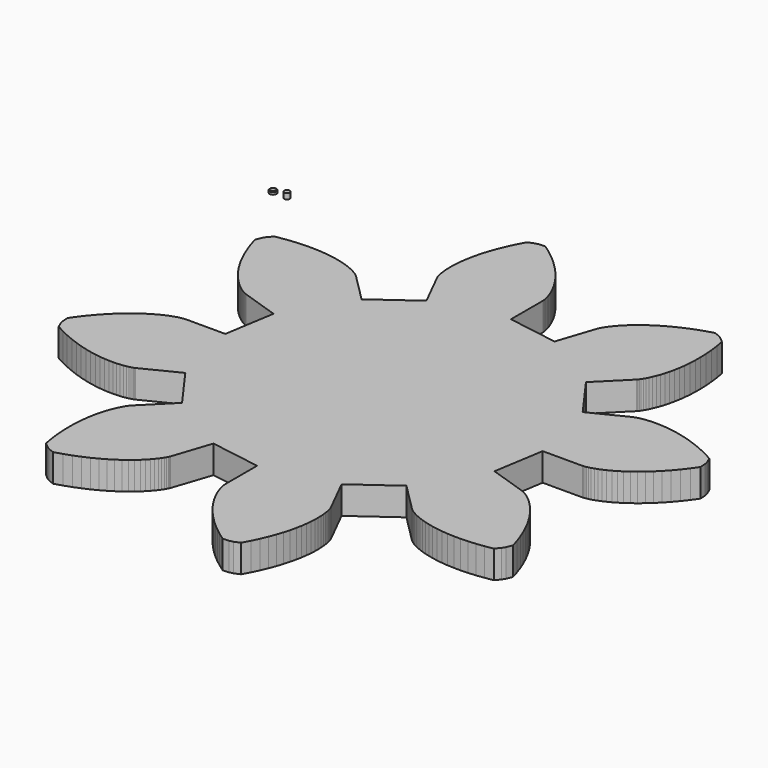
from build123d import *

# Parameters (mm, degrees)
F0_R     = 31.75
F0_R_2   = 25.4
F1_DEPTH = 25.4
F0_R_3   = 25.4571162214
F2_DEPTH = 50.8
F3_R     = 2.54
F6_DEPTH = 254


# Not quite as in the source:
# - a fillet or chamfer that OpenCascade refuses, or shapes differently, is made with other operations: its cross-section is extruded or revolved along the edge and cut away or added


with BuildPart() as f1:
    # F0 (on Top) → F1 (new body)
    with BuildSketch(Plane.XY):
        with Locations((-25.4, 10.8899995685)):
            Circle(F0_R)
        with Locations((-25.4, 10.8899995685)):
            Circle(F0_R_2, mode=Mode.SUBTRACT)
    extrude(amount=F1_DEPTH)

    # F3
    f3_edges = [f1.edges().sort_by_distance(p)[0] for p in [
        (-50.8, 10.89, 25.4),
    ]]
    fillet(f3_edges, radius=F3_R)

    # F4: chamfer of 5.08 on 1 edges, made by hand

    # F4_s1 → F4_t2 (revolve, cut)
    with BuildSketch(Plane.XZ.offset(-10.8899995685)):
        Polygon((1.27, 25.4), (6.35, 20.32), (6.35, 25.4), align=None)
    revolve(axis=Axis((-25.4, 10.8899995685, 25.4), (0, 0, 1)), mode=Mode.SUBTRACT)


with BuildPart() as f2:
    # F0 (on Top) → F2 (new body)
    with BuildSketch(Plane.XY):
        with Locations((101.6, 10.8899995685)):
            Circle(F0_R_3)
    extrude(amount=F2_DEPTH)


with BuildPart() as f6:
    # F5 (on face) → F6 (new body)
    with BuildSketch(Plane.XY.offset(50.8)):
        Polygon((4697.3145576, -2359.8523288), (4703.8413416, -2359.2975928), (4713.7554696, -2358.0235288), (4727.0000456, -2355.7354968), (4743.5019176, -2352.1408888), (4763.1635496, -2346.9511608), (4785.8731816, -2339.8858968), (4811.4967016, -2330.6728088), (4839.8837416, -2319.0457048), (4870.8656456, -2304.7485528), (4904.2595336, -2287.5354808), (4939.8642376, -2267.1728088), (4977.4603016, -2243.4349848), (5016.8181096, -2216.1167768), (5057.6897576, -2185.0210808), (5099.8151496, -2149.9690808), (5142.9240296, -2110.7941528), (5186.7319176, -2067.3520248), (5230.9421416, -2019.5065528), (5275.2499016, -1967.1480088), (5319.3422696, -1910.1829208), (5362.8961576, -1848.5340728), (5359.2670056, -1792.7556728), (5351.1227496, -1758.3092088), (5329.3864456, -1706.8142648), (5262.8323496, -1671.1994008), (5197.8977576, -1640.0122648), (5134.8326056, -1613.0435608), (5073.8766696, -1590.0657048), (5015.2514376, -1570.8429848), (4959.1641736, -1555.1234328), (4905.7997896, -1542.6489848), (4855.3289736, -1533.1514168), (4807.9041256, -1526.3543768), (4763.6593576, -1521.9693208), (4722.7043976, -1519.7077048), (4685.1388136, -1519.2728568), (4651.0337256, -1520.3660728), (4620.4460296, -1522.6845848), (4593.4102696, -1525.9215608), (4569.9427016, -1529.7762648), (4550.0372296, -1533.9418648), (4533.6735336, -1538.1176248), (4520.8048776, -1542.0048408), (4511.3703016, -1545.3048088), (4505.2864936, -1547.7310168), (4502.4559176, -1548.9989848), (4177.8947176, -1711.5711768), (3907.1652616, -1336.2404568), (4163.8434376, -1079.5582168), (4165.9384296, -1077.2722168), (4170.1609256, -1072.2653688), (4176.2711496, -1064.3547928), (4184.0171336, -1053.3698008), (4193.1448776, -1039.1600248), (4203.3780296, -1021.5872888), (4214.4402376, -1000.5337368), (4226.0429576, -975.8998008), (4237.8956136, -947.6062328), (4249.6934056, -915.5880088), (4261.1355976, -879.8044888), (4271.9112936, -840.2292568), (4281.7116296, -796.8602808), (4290.2257096, -749.7138168), (4297.1385736, -698.8244088), (4302.1393256, -644.2509848), (4304.9211336, -586.0687288), (4305.1791976, -524.3731448), (4302.6087176, -459.2800568), (4296.9170856, -390.9276408), (4287.8137256, -319.4682968), (4275.0182216, -245.0788088), (4233.0106856, -208.2020728), (4202.8964456, -189.6052088), (4151.1109256, -168.5618168), (4078.8692616, -190.4383288), (4010.9008936, -214.3041688), (3947.2363016, -239.8260888), (3887.8856456, -266.6810008), (3832.8387656, -294.5417528), (3782.0631496, -323.0872888), (3735.5100296, -352.0026488), (3693.1062536, -380.9749048), (3654.7644456, -409.7012888), (3620.3769096, -437.8871608), (3589.8196936, -465.2460088), (3562.9485256, -491.5035128), (3539.6069416, -516.3914488), (3519.6161256, -539.6598808), (3502.7891336, -561.0670008), (3488.9187016, -580.3852248), (3477.7914696, -597.4072888), (3469.1717256, -611.9299928), (3462.8196936, -623.7785848), (3458.4834056, -632.7823768), (3455.8987016, -638.7991288), (3454.7932936, -641.6987928), (3340.2494536, -986.1532728), (2883.4152136, -912.1905048), (2883.4111496, -549.1899608), (2883.2689096, -546.0911608), (2882.7141736, -539.5643768), (2881.4401096, -529.6502488), (2879.1520776, -516.4056728), (2875.5574696, -499.9038008), (2870.3677416, -480.2421688), (2863.3024776, -457.5325368), (2854.0893896, -431.9090168), (2842.4622856, -403.5219768), (2828.1651336, -372.5400728), (2810.9520616, -339.1461848), (2790.5893896, -303.5414808), (2766.8515656, -265.9454168), (2739.5333576, -226.5876088), (2708.4376616, -185.7159608), (2673.3856616, -143.5905688), (2634.2107336, -100.4816888), (2590.7686056, -56.6738008), (2542.9231336, -12.4635768), (2490.5645896, 31.8441832), (2433.5995016, 75.9365512), (2371.9506536, 119.4904392), (2316.1722536, 115.8612872), (2281.7257896, 107.7170312), (2230.2308456, 85.9807272), (2194.6159816, 19.4266312), (2163.4288456, -45.5079608), (2136.4601416, -108.5731128), (2113.4822856, -169.5290488), (2094.2595656, -228.1542808), (2078.5400136, -284.2415448), (2066.0655656, -337.6059288), (2056.5679976, -388.0767448), (2049.7709576, -435.5015928), (2045.3859016, -479.7463608), (2043.1242856, -520.7013208), (2042.6894376, -558.2669048), (2043.7826536, -592.3719928), (2046.1011656, -622.9596888), (2049.3381416, -649.9954488), (2053.1928456, -673.4630168), (2057.3584456, -693.3684888), (2061.5342056, -709.7321848), (2065.4214216, -722.6008408), (2068.7213896, -732.0354168), (2071.1475976, -738.1192248), (2072.4155656, -740.9498008), (2234.9877576, -1065.5110008), (1859.6570376, -1336.2404568), (1602.9747976, -1079.5622808), (1600.6887976, -1077.4672888), (1595.6819496, -1073.2447928), (1587.7713736, -1067.1345688), (1576.7863816, -1059.3885848), (1562.5766056, -1050.2608408), (1545.0038696, -1040.0276888), (1523.9503176, -1028.9654808), (1499.3163816, -1017.3627608), (1471.0228136, -1005.5101048), (1439.0045896, -993.7123128), (1403.2210696, -982.2701208), (1363.6458376, -971.4944248), (1320.2768616, -961.6940888), (1273.1303976, -953.1800088), (1222.2409896, -946.2671448), (1167.6675656, -941.2663928), (1109.4853096, -938.4845848), (1047.7897256, -938.2265208), (982.6966376, -940.7970008), (914.3442216, -946.4886328), (842.8848776, -955.5919928), (768.4953896, -968.3874968), (731.6186536, -1010.3950328), (713.0217896, -1040.5092728), (691.9783976, -1092.2947928), (713.8549096, -1164.5364568), (737.7207496, -1232.5048248), (763.2426696, -1296.1694168), (790.0975816, -1355.5200728), (817.9583336, -1410.5669528), (846.5038696, -1461.3425688), (875.4192296, -1507.8956888), (904.3914856, -1550.2994648), (933.1178696, -1588.6412728), (961.3037416, -1623.0288088), (988.6625896, -1653.5860248), (1014.9200936, -1680.4571928), (1039.8080296, -1703.7987768), (1063.0764616, -1723.7895928), (1084.4835816, -1740.6165848), (1103.8018056, -1754.4870168), (1120.8238696, -1765.6142488), (1135.3465736, -1774.2339928), (1147.1951656, -1780.5860248), (1156.1989576, -1784.9223128), (1162.2157096, -1787.5070168), (1165.1153736, -1788.6124248), (1509.5698536, -1903.1562648), (1435.6070856, -2359.9905048), (1072.6065416, -2359.9945688), (1069.5077416, -2360.1368088), (1062.9809576, -2360.6915448), (1053.0668296, -2361.9656088), (1039.8222536, -2364.2536408), (1023.3203816, -2367.8482488), (1003.6587496, -2373.0379768), (980.9491176, -2380.1032408), (955.3255976, -2389.3163288), (926.9385576, -2400.9434328), (895.9566536, -2415.2405848), (862.5627656, -2432.4536568), (826.9580616, -2452.8163288), (789.3619976, -2476.5541528), (750.0041896, -2503.8723608), (709.1325416, -2534.9680568), (667.0071496, -2570.0200568), (623.8982696, -2609.1949848), (580.0903816, -2652.6371128), (535.8801576, -2700.4825848), (491.5723976, -2752.8411288), (447.4800296, -2809.8062168), (403.9261416, -2871.4550648), (407.5552936, -2927.2334648), (415.6995496, -2961.6799288), (437.4358536, -3013.1748728), (503.9899496, -3048.7897368), (568.9245416, -3079.9768728), (631.9896936, -3106.9455768), (692.9456296, -3129.9234328), (751.5708616, -3149.1461528), (807.6581256, -3164.8657048), (861.0225096, -3177.3401528), (911.4933256, -3186.8377208), (958.9181736, -3193.6347608), (1003.1629416, -3198.0198168), (1044.1179016, -3200.2814328), (1081.6834856, -3200.7162808), (1115.7885736, -3199.6230648), (1146.3762696, -3197.3045528), (1173.4120296, -3194.0675768), (1196.8795976, -3190.2128728), (1216.7850696, -3186.0472728), (1233.1487656, -3181.8715128), (1246.0174216, -3177.9842968), (1255.4519976, -3174.6843288), (1261.5358056, -3172.2581208), (1264.3663816, -3170.9901528), (1588.9275816, -3008.4179608), (1859.6570376, -3383.7486808), (1602.9788616, -3640.4309208), (1600.8838696, -3642.7169208), (1596.6613736, -3647.7237688), (1590.5511496, -3655.6343448), (1582.8051656, -3666.6193368), (1573.6774216, -3680.8291128), (1563.4442696, -3698.4018488), (1552.3820616, -3719.4554008), (1540.7793416, -3744.0893368), (1528.9266856, -3772.3829048), (1517.1288936, -3804.4011288), (1505.6867016, -3840.1846488), (1494.9110056, -3879.7598808), (1485.1106696, -3923.1288568), (1476.5965896, -3970.2753208), (1469.6837256, -4021.1647288), (1464.6829736, -4075.7381528), (1461.9011656, -4133.9204088), (1461.6431016, -4195.6159928), (1464.2135816, -4260.7090808), (1469.9052136, -4329.0614968), (1479.0085736, -4400.5208408), (1491.8040776, -4474.9103288), (1533.8116136, -4511.7870648), (1563.9258536, -4530.3839288), (1615.7113736, -4551.4273208), (1687.9530376, -4529.5508088), (1755.9214056, -4505.6849688), (1819.5859976, -4480.1630488), (1878.9366536, -4453.3081368), (1933.9835336, -4425.4473848), (1984.7591496, -4396.9018488), (2031.3122696, -4367.9864888), (2073.7160456, -4339.0142328), (2112.0578536, -4310.2878488), (2146.4453896, -4282.1019768), (2177.0026056, -4254.7431288), (2203.8737736, -4228.4856248), (2227.2153576, -4203.5976888), (2247.2061736, -4180.3292568), (2264.0331656, -4158.9221368), (2277.9035976, -4139.6039128), (2289.0308296, -4122.5818488), (2297.6505736, -4108.0591448), (2304.0026056, -4096.2105528), (2308.3388936, -4087.2067608), (2310.9235976, -4081.1900088), (2312.0290056, -4078.2903448), (2426.5728456, -3733.8358648), (2883.4070856, -3807.7986328), (2883.4111496, -4170.7991768), (2883.5533896, -4173.8979768), (2884.1081256, -4180.4247608), (2885.3821896, -4190.3388888), (2887.6702216, -4203.5834648), (2891.2648296, -4220.0853368), (2896.4545576, -4239.7469688), (2903.5198216, -4262.4566008), (2912.7329096, -4288.0801208), (2924.3600136, -4316.4671608), (2938.6571656, -4347.4490648), (2955.8702376, -4380.8429528), (2976.2329096, -4416.4476568), (2999.9707336, -4454.0437208), (3027.2889416, -4493.4015288), (3058.3846376, -4534.2731768), (3093.4366376, -4576.3985688), (3132.6115656, -4619.5074488), (3176.0536936, -4663.3153368), (3223.8991656, -4707.5255608), (3276.2577096, -4751.8333208), (3333.2227976, -4795.9256888), (3394.8716456, -4839.4795768), (3450.6500456, -4835.8504248), (3485.0965096, -4827.7061688), (3536.5914536, -4805.9698648), (3572.2063176, -4739.4157688), (3603.3934536, -4674.4811768), (3630.3621576, -4611.4160248), (3653.3400136, -4550.4600888), (3672.5627336, -4491.8348568), (3688.2822856, -4435.7475928), (3700.7567336, -4382.3832088), (3710.2543016, -4331.9123928), (3717.0513416, -4284.4875448), (3721.4363976, -4240.2427768), (3723.6980136, -4199.2878168), (3724.1328616, -4161.7222328), (3723.0396456, -4127.6171448), (3720.7211336, -4097.0294488), (3717.4841576, -4069.9936888), (3713.6294536, -4046.5261208), (3709.4638536, -4026.6206488), (3705.2880936, -4010.2569528), (3701.4008776, -3997.3882968), (3698.1009096, -3987.9537208), (3695.6747016, -3981.8699128), (3694.4067336, -3979.0393368), (3531.8345416, -3654.4781368), (3907.1652616, -3383.7486808), (4163.8475016, -3640.4268568), (4166.1335016, -3642.5218488), (4171.1403496, -3646.7443448), (4179.0509256, -3652.8545688), (4190.0359176, -3660.6005528), (4204.2456936, -3669.7282968), (4221.8184296, -3679.9614488), (4242.8719816, -3691.0236568), (4267.5059176, -3702.6263768), (4295.7994856, -3714.4790328), (4327.8177096, -3726.2768248), (4363.6012296, -3737.7190168), (4403.1764616, -3748.4947128), (4446.5454376, -3758.2950488), (4493.6919016, -3766.8091288), (4544.5813096, -3773.7219928), (4599.1547336, -3778.7227448), (4657.3369896, -3781.5045528), (4719.0325736, -3781.7626168), (4784.1256616, -3779.1921368), (4852.4780776, -3773.5005048), (4923.9374216, -3764.3971448), (4998.3269096, -3751.6016408), (5035.2036456, -3709.5941048), (5053.8005096, -3679.4798648), (5074.8439016, -3627.6943448), (5052.9673896, -3555.4526808), (5029.1015496, -3487.4843128), (5003.5796296, -3423.8197208), (4976.7247176, -3364.4690648), (4948.8639656, -3309.4221848), (4920.3184296, -3258.6465688), (4891.4030696, -3212.0934488), (4862.4308136, -3169.6896728), (4833.7044296, -3131.3478648), (4805.5185576, -3096.9603288), (4778.1597096, -3066.4031128), (4751.9022056, -3039.5319448), (4727.0142696, -3016.1903608), (4703.7458376, -2996.1995448), (4682.3387176, -2979.3725528), (4663.0204936, -2965.5021208), (4645.9984296, -2954.3748888), (4631.4757256, -2945.7551448), (4619.6271336, -2939.4031128), (4610.6233416, -2935.0668248), (4604.6065896, -2932.4821208), (4601.7069256, -2931.3767128), (4257.2524456, -2816.8328728), (4331.2152136, -2359.9986328), (4694.2157576, -2359.9945688), align=None)
    extrude(amount=F6_DEPTH)


solid = Compound([f1.part, f2.part, f6.part])
